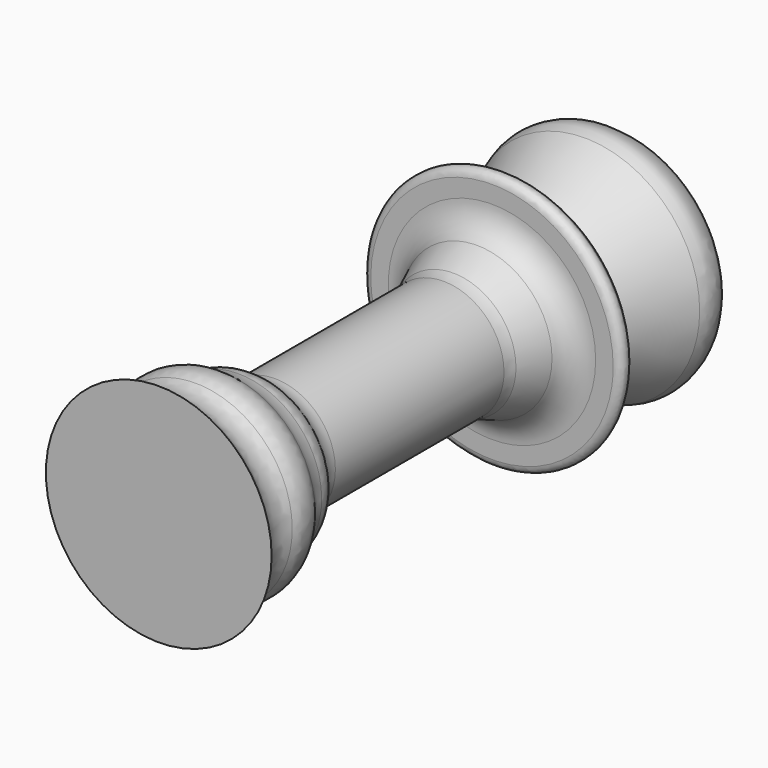
from build123d import *

# Parameters (mm, degrees)
F2_R  = 5.08
F4_R  = 5.08
F6_R  = 5.08
F7_R  = 5.08
F8_R  = 5.08
F9_R  = 1.27
F10_R = 5.08


# Not quite as in the source:
# - a fillet or chamfer that OpenCascade refuses, or shapes differently, is made with other operations: its cross-section is extruded or revolved along the edge and cut away or added


with BuildPart() as f1:
    # F0 (on Top) → F1 (revolve)
    with BuildSketch(Plane.XY):
        Polygon((0, 44.4659888744), (0, -53.1001612544), (18.5634717345, -53.1001612544), (13.6707723141, -48.207461834), (18.5634717345, -43.3147624135), (13.6707723141, -38.422062993), (13.6707723141, -34.1049805284), (9.9292984232, -34.1049805284), (9.9292984232, 6.4756297506), (13.6707723141, 15.3976073489), (21.7293351889, 15.3976073489), (21.7293351889, 19.7146944702), (13.6707723141, 19.7146944702), (13.6707723141, 23.4561692923), (21.7293351889, 40.4367111623), align=None)
    revolve(axis=Axis((0, -4.31708619, 0), (0, -1, 0)))

    # F2
    f2_edges = [f1.edges().sort_by_distance(p)[0] for p in [
        (-21.729335, 40.436711, 0),
    ]]
    fillet(f2_edges, radius=F2_R)

    # F3: fillet of radius 5.08 on 1 edges, made by hand

    # F3_s1 → F3_t2 (revolve, cut)
    with BuildSketch(Plane.XY):
        with BuildLine():
            ThreePointArc((16.7069489095, 19.7146944702), (20.0183536398, 18.4870961512), (21.7293351889, 15.3976073489))
            Line((21.7293351889, 15.3976073489), (21.7293351889, 19.7146944702))
            Line((21.7293351889, 19.7146944702), (16.7069489095, 19.7146944702))
        make_face()
    revolve(axis=Axis((0, 19.7146944702, 0), (0, -1, 0)), mode=Mode.SUBTRACT)

    # F4
    f4_edges = [f1.edges().sort_by_distance(p)[0] for p in [
        (-9.929298, 6.47563, 0),
        (-13.670772, 15.397607, 0),
        (11.800035, 10.936619, 0),
    ]]
    fillet(f4_edges, radius=F4_R)

    # F5: fillet of radius 5.08 on 3 edges, made by hand

    # F5_s1 → F5_t2 (revolve)
    with BuildSketch(Plane.XY):
        with BuildLine():
            ThreePointArc((9.9292984232, -29.2044960773), (10.9715940857, -32.287245448), (13.6707723141, -34.1049805284))
            Line((13.6707723141, -34.1049805284), (9.9292984232, -34.1049805284))
            Line((9.9292984232, -34.1049805284), (9.9292984232, -29.2044960773))
        make_face()
    revolve(axis=Axis((0, -34.1049805284, 0), (0, -1, 0)))

    # F6
    f6_edges = [f1.edges().sort_by_distance(p)[0] for p in [
        (-18.563472, -43.314762, 0),
    ]]
    fillet(f6_edges, radius=F6_R)

    # F7
    f7_edges = [f1.edges().sort_by_distance(p)[0] for p in [
        (-13.670772, -38.422063, 0),
    ]]
    fillet(f7_edges, radius=F7_R)

    # F8
    f8_edges = [f1.edges().sort_by_distance(p)[0] for p in [
        (-13.670772, -48.207462, 0),
    ]]
    fillet(f8_edges, radius=F8_R)

    # F9
    f9_edges = [f1.edges().sort_by_distance(p)[0] for p in [
        (-21.729335, 15.397607, 0),
    ]]
    fillet(f9_edges, radius=F9_R)

    # F10
    f10_edges = [f1.edges().sort_by_distance(p)[0] for p in [
        (-13.670772, -34.104981, 0),
    ]]
    fillet(f10_edges, radius=F10_R)


solid = f1.part
